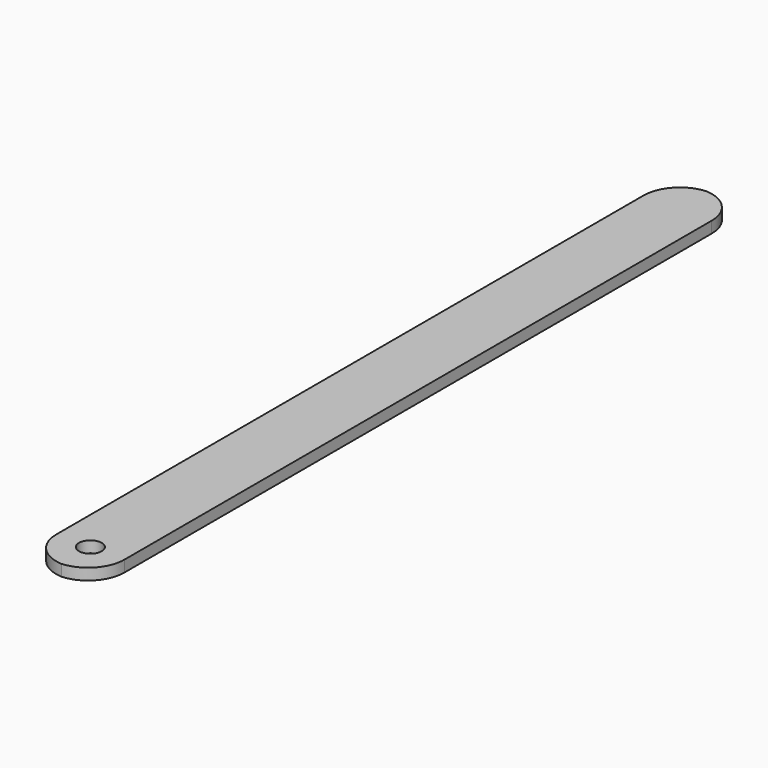
from build123d import *

# Parameters (mm, degrees)
F0_W        = 9.525
F0_H        = 112.7125
F1_DEPTH    = 1.5875
F2_T1_DEPTH = 26.9875
F4_D        = 3.175


# Not quite as in the source:
# - a fillet or chamfer that OpenCascade refuses, or shapes differently, is made with other operations: its cross-section is extruded or revolved along the edge and cut away or added


with BuildPart() as f1:
    # F0 (on Top) → F1 (new body)
    with BuildSketch(Plane.XY):
        with Locations((0, 56.35625)):
            Rectangle(F0_W, F0_H)
    extrude(amount=F1_DEPTH)

    # F2: fillet of radius 5.08 on 4 edges, made by hand

    # F2_s2 → F2_t1 (cut)
    with BuildSketch(Plane.XY.offset(-12.7)):
        with BuildLine():
            ThreePointArc((-0.3175, 0), (3.2746024484, 1.4878975516), (4.7625, 5.08))
            Line((4.7625, 5.08), (4.7625, 0))
            Line((4.7625, 0), (-0.3175, 0))
        make_face()
        with BuildLine():
            ThreePointArc((-4.7625, 5.08), (-3.2746024484, 1.4878975516), (0.3175, 0))
            Line((0.3175, 0), (-4.7625, 0))
            Line((-4.7625, 0), (-4.7625, 5.08))
        make_face()
        with BuildLine():
            ThreePointArc((-0.3175, 112.7125), (3.2746024484, 111.2246024484), (4.7625, 107.6325))
            Line((4.7625, 107.6325), (4.7625, 112.7125))
            Line((4.7625, 112.7125), (-0.3175, 112.7125))
        make_face()
        with BuildLine():
            ThreePointArc((0.3175, 112.7125), (-3.2746024484, 111.2246024484), (-4.7625, 107.6325))
            Line((-4.7625, 107.6325), (-4.7625, 112.7125))
            Line((-4.7625, 112.7125), (0.3175, 112.7125))
        make_face()
    extrude(amount=F2_T1_DEPTH, mode=Mode.SUBTRACT)

    # F4 (through all)
    with Locations(Plane.XY.offset(1.5875)):
        with Locations((0, 5.08)):
            Hole(F4_D / 2)


solid = f1.part
